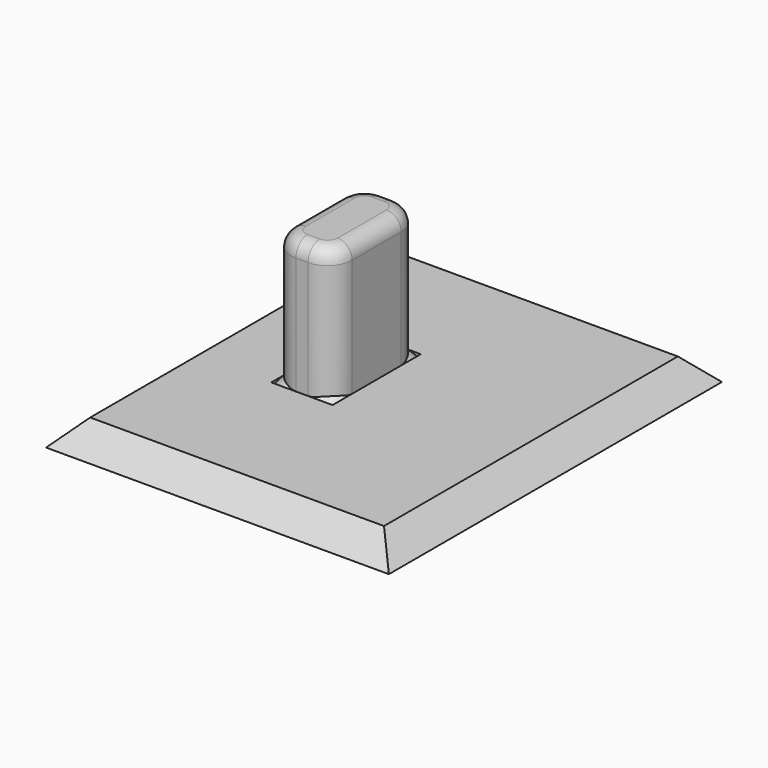
from build123d import *

# Parameters (mm, degrees)
F0_W         = 70
F0_H         = 85
F0_W_2       = 12.5
F0_H_2       = 22.5
F1_DEPTH     = 5
F2_SIZE      = 4.99999
F3_DEPTH     = 32
F4_R         = 3
F5_T1_DEPTH  = 44.5
F5_T4_ANGLE  = 90
F5_T6_ANGLE  = 90
F5_T8_ANGLE  = 90
F5_T10_ANGLE = 90
F6_DEPTH     = 10
F7_SIZE      = 5
F8_T1_DEPTH  = 23.0940107676
F8_T3_DEPTH  = 23.0940107676
F8_T5_DEPTH  = 23.0940107676
F8_T7_DEPTH  = 23.0940107676


# Not quite as in the source:
# - a fillet or chamfer that OpenCascade refuses, or shapes differently, is made with other operations: its cross-section is extruded or revolved along the edge and cut away or added
# - a fillet or chamfer is up to 0.001 mm smaller than in the source, because OpenCascade refuses the exact size


with BuildPart() as f1:
    # F0 (on Top) → F1 (new body)
    with BuildSketch(Plane.XY):
        with Locations((1.3024921715, 25.2146533675)):
            Rectangle(F0_W, F0_H)
        with Locations((-7.4475078285, 26.4646533675)):
            Rectangle(F0_W_2, F0_H_2, mode=Mode.SUBTRACT)
    extrude(amount=F1_DEPTH)

    # F2 (size 5 in the source; OpenCascade refuses exactly that, so slightly less here)
    f2_edges = [f1.edges().sort_by_distance(p)[0] for p in [
        (-33.697508, 25.214653, 5),
        (1.302492, -17.285347, 5),
        (36.302492, 25.214653, 5),
        (1.302492, 67.714653, 5),
    ]]
    chamfer(f2_edges, length=F2_SIZE)


with BuildPart() as f3:
    # F0 (on Top) → F3 (new body)
    with BuildSketch(Plane.XY):
        with Locations((-7.4475078285, 26.4646533675)):
            Rectangle(F0_W_2, F0_H_2)
    extrude(amount=F3_DEPTH)

    # F4
    f4_edges = [f3.edges().sort_by_distance(p)[0] for p in [
        (-13.697508, 26.464653, 32),
        (-7.447508, 15.214653, 32),
        (-7.447508, 37.714653, 32),
        (-1.197508, 26.464653, 32),
    ]]
    fillet(f4_edges, radius=F4_R)

    # F5: fillet of radius 5 on 8 edges, made by hand

    # F5_s2 → F5_t1 (cut)
    with BuildSketch(Plane.XY.offset(-12.5)):
        with BuildLine():
            ThreePointArc((-1.1975078285, 32.7146533675), (-2.6619739225, 36.2501872734), (-6.1975078285, 37.7146533675))
            Line((-6.1975078285, 37.7146533675), (-1.1975078285, 37.7146533675))
            Line((-1.1975078285, 37.7146533675), (-1.1975078285, 32.7146533675))
        make_face()
        with BuildLine():
            ThreePointArc((-6.1975078285, 15.2146533675), (-2.6619739225, 16.6791194616), (-1.1975078285, 20.2146533675))
            Line((-1.1975078285, 20.2146533675), (-1.1975078285, 15.2146533675))
            Line((-1.1975078285, 15.2146533675), (-6.1975078285, 15.2146533675))
        make_face()
        with BuildLine():
            ThreePointArc((-8.6975078285, 15.2146533675), (-12.2330417344, 16.6791194616), (-13.6975078285, 20.2146533675))
            Line((-13.6975078285, 20.2146533675), (-13.6975078285, 15.2146533675))
            Line((-13.6975078285, 15.2146533675), (-8.6975078285, 15.2146533675))
        make_face()
        with BuildLine():
            ThreePointArc((-13.6975078285, 32.7146533675), (-12.2330417344, 36.2501872734), (-8.6975078285, 37.7146533675))
            Line((-8.6975078285, 37.7146533675), (-13.6975078285, 37.7146533675))
            Line((-13.6975078285, 37.7146533675), (-13.6975078285, 32.7146533675))
        make_face()
    extrude(amount=F5_T1_DEPTH, mode=Mode.SUBTRACT)

    # F5_s3 → F5_t4 (revolve, cut)
    with BuildSketch(Plane.YZ.offset(-8.6975078285)):
        with BuildLine():
            ThreePointArc((34.7146533675, 32), (36.8359737111, 31.1213203436), (37.7146533675, 29))
            Line((37.7146533675, 29), (37.7146533675, 32))
            Line((37.7146533675, 32), (34.7146533675, 32))
        make_face()
    revolve(axis=Axis((-8.6975078285, 32.7146533675, 32), (0, 0, 1)), revolution_arc=F5_T4_ANGLE, mode=Mode.SUBTRACT)

    # F5_s5 → F5_t6 (revolve, cut)
    with BuildSketch(Plane.XZ.offset(-20.2146533675)):
        with BuildLine():
            ThreePointArc((-10.6975078285, 32), (-12.818828172, 31.1213203436), (-13.6975078285, 29))
            Line((-13.6975078285, 29), (-13.6975078285, 32))
            Line((-13.6975078285, 32), (-10.6975078285, 32))
        make_face()
    revolve(axis=Axis((-8.6975078285, 20.2146533675, 32), (0, 0, 1)), revolution_arc=F5_T6_ANGLE, mode=Mode.SUBTRACT)

    # F5_s7 → F5_t8 (revolve, cut)
    with BuildSketch(Plane.YZ.offset(-6.1975078285)):
        with BuildLine():
            ThreePointArc((18.2146533675, 32), (16.0933330239, 31.1213203436), (15.2146533675, 29))
            Line((15.2146533675, 29), (15.2146533675, 32))
            Line((15.2146533675, 32), (18.2146533675, 32))
        make_face()
    revolve(axis=Axis((-6.1975078285, 20.2146533675, 32), (0, 0, 1)), revolution_arc=F5_T8_ANGLE, mode=Mode.SUBTRACT)

    # F5_s9 → F5_t10 (revolve, cut)
    with BuildSketch(Plane.XZ.offset(-32.7146533675)):
        with BuildLine():
            ThreePointArc((-4.1975078285, 32), (-2.0761874849, 31.1213203436), (-1.1975078285, 29))
            Line((-1.1975078285, 29), (-1.1975078285, 32))
            Line((-1.1975078285, 32), (-4.1975078285, 32))
        make_face()
    revolve(axis=Axis((-6.1975078285, 32.7146533675, 32), (0, 0, 1)), revolution_arc=F5_T10_ANGLE, mode=Mode.SUBTRACT)


with BuildPart() as f6:
    # F0 (on Top) → F6 (new body)
    with BuildSketch(Plane.XY):
        with Locations((-7.4475078285, 26.4646533675)):
            Rectangle(F0_W_2, F0_H_2)
    extrude(amount=F6_DEPTH)

    # F7
    f7_edges = [f6.edges().sort_by_distance(p)[0] for p in [
        (-13.697508, 26.464653, 10),
        (-7.447508, 15.214653, 10),
        (-1.197508, 26.464653, 10),
        (-7.447508, 37.714653, 10),
    ]]
    chamfer(f7_edges, length=F7_SIZE)

    # F8: fillet of radius 5 on 4 edges, made by hand

    # F8_s2 → F8_t1 (cut)
    with BuildSketch(Plane(origin=(-19.6373870653, 19.6373870653, -19.6373870653), x_dir=(0.7071067812, 0.7071067812, 0), z_dir=(0.5773502692, -0.5773502692, 0.5773502692))):
        with BuildLine():
            ThreePointArc((14.4826864754, 23.628034149), (16.9826864754, 24.2979071301), (19.4826864754, 23.628034149))
            Line((19.4826864754, 23.628034149), (16.9826864754, 25.0714098219))
            Line((16.9826864754, 25.0714098219), (14.4826864754, 23.628034149))
        make_face()
    extrude(amount=F8_T1_DEPTH, mode=Mode.SUBTRACT)

    # F8_s4 → F8_t3 (cut)
    with BuildSketch(Plane(origin=(14.6723818463, 14.6723818463, -14.6723818463), x_dir=(0.7071067812, -0.7071067812, 0), z_dir=(-0.5773502692, -0.5773502692, 0.5773502692))):
        with BuildLine():
            ThreePointArc((-25.0150530523, 17.5471694706), (-27.5150530523, 18.2170424517), (-30.0150530523, 17.5471694706))
            Line((-30.0150530523, 17.5471694706), (-27.5150530523, 18.9905451436))
            Line((-27.5150530523, 18.9905451436), (-25.0150530523, 17.5471694706))
        make_face()
    extrude(amount=F8_T3_DEPTH, mode=Mode.SUBTRACT)

    # F8_s6 → F8_t5 (cut)
    with BuildSketch(Plane(origin=(-1.9942848203, -1.9942848203, -1.9942848203), x_dir=(-0.7071067812, 0.7071067812, 0), z_dir=(0.5773502692, 0.5773502692, 0.5773502692))):
        with BuildLine():
            ThreePointArc((17.9439852404, 2.019735159), (20.4439852404, 2.68960814), (22.9439852404, 2.019735159))
            Line((22.9439852404, 2.019735159), (20.4439852404, 3.4631108319))
            Line((20.4439852404, 3.4631108319), (17.9439852404, 2.019735159))
        make_face()
    extrude(amount=F8_T5_DEPTH, mode=Mode.SUBTRACT)

    # F8_s8 → F8_t7 (cut)
    with BuildSketch(Plane(origin=(-2.9707203987, 2.9707203987, 2.9707203987), x_dir=(-0.7071067812, -0.7071067812, 0), z_dir=(-0.5773502692, 0.5773502692, 0.5773502692))):
        with BuildLine():
            ThreePointArc((-7.4116186635, -4.0611295194), (-9.9116186635, -3.3912565383), (-12.4116186635, -4.0611295194))
            Line((-12.4116186635, -4.0611295194), (-9.9116186635, -2.6177538464))
            Line((-9.9116186635, -2.6177538464), (-7.4116186635, -4.0611295194))
        make_face()
    extrude(amount=F8_T7_DEPTH, mode=Mode.SUBTRACT)


solid = Compound([f1.part, f3.part, f6.part])
